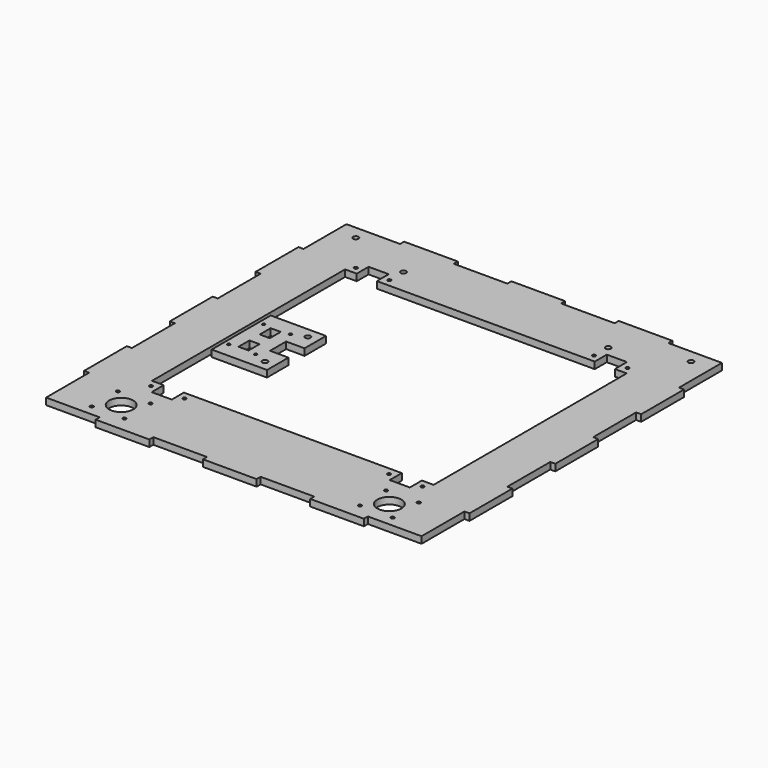
from build123d import *

# Parameters (mm, degrees)
F0_R     = 1.5875
F0_R_2   = 11.43
F0_R_3   = 3.175
F0_W     = 4.7625
F0_H     = 50.8
F0_W_2   = 50.8
F0_H_2   = 4.7625
F0_W_3   = 44.45
F0_H_3   = 41.1268851364
F1_DEPTH = 6.35
F0_R_4   = 1.8415
F0_W_4   = 9.525
F0_H_4   = 12.954
F2_D     = 2.7051
F3_D     = 5.1054
F4_D     = 5.1054


with BuildPart() as f1:
    # F0 (on Top) → F1 (new body)
    with BuildSketch(Plane.XY):
        with BuildLine():
            ThreePointArc((155.575, 171.45), (158.75, 174.625), (161.925, 171.45))
            Line((161.925, 171.45), (177.8, 171.45))
            Line((177.8, 171.45), (177.8, 184.15))
            Line((177.8, 184.15), (127, 184.15))
            Line((127, 184.15), (76.2, 184.15))
            Line((76.2, 184.15), (25.4, 184.15))
            Line((25.4, 184.15), (-25.4, 184.15))
            Line((-25.4, 184.15), (-76.2, 184.15))
            Line((-76.2, 184.15), (-127, 184.15))
            Line((-127, 184.15), (-177.8, 184.15))
            Line((-177.8, 184.15), (-177.8, 171.45))
            Line((-177.8, 171.45), (-161.925, 171.45))
            ThreePointArc((-161.925, 171.45), (-158.75, 174.625), (-155.575, 171.45))
            Line((-155.575, 171.45), (155.575, 171.45))
        make_face()
        with BuildLine():
            ThreePointArc((155.575, 171.45), (158.75, 168.275), (161.925, 171.45))
            Line((161.925, 171.45), (155.575, 171.45))
        make_face()
        with BuildLine():
            Line((155.575, 171.45), (161.925, 171.45))
            ThreePointArc((161.925, 171.45), (158.75, 174.625), (155.575, 171.45))
        make_face()
        with BuildLine():
            Line((177.8, 171.45), (161.925, 171.45))
            ThreePointArc((161.925, 171.45), (158.75, 168.275), (155.575, 171.45))
            Line((155.575, 171.45), (-155.575, 171.45))
            ThreePointArc((-155.575, 171.45), (-158.75, 168.275), (-161.925, 171.45))
            Line((-161.925, 171.45), (-177.8, 171.45))
            Line((-177.8, 171.45), (-177.8, 133.35))
            Line((-177.8, 133.35), (-177.8, 82.55))
            Line((-177.8, 82.55), (-177.8, 31.75))
            Line((-177.8, 31.75), (-177.8, -19.05))
            Line((-177.8, -19.05), (-177.8, -69.85))
            Line((-177.8, -69.85), (-177.8, -120.65))
            Line((-177.8, -120.65), (-177.8, -171.45))
            Line((-177.8, -171.45), (-127, -171.45))
            Line((-127, -171.45), (-76.2, -171.45))
            Line((-76.2, -171.45), (-25.4, -171.45))
            Line((-25.4, -171.45), (25.4, -171.45))
            Line((25.4, -171.45), (76.2, -171.45))
            Line((76.2, -171.45), (127, -171.45))
            Line((127, -171.45), (177.8, -171.45))
            Line((177.8, -171.45), (177.8, -120.65))
            Line((177.8, -120.65), (177.8, -69.85))
            Line((177.8, -69.85), (177.8, -19.05))
            Line((177.8, -19.05), (177.8, 31.75))
            Line((177.8, 31.75), (177.8, 82.55))
            Line((177.8, 82.55), (177.8, 133.35))
            Line((177.8, 133.35), (177.8, 171.45))
        make_face()
        with Locations((-142.494, -161.544)):
            Circle(F0_R, mode=Mode.SUBTRACT)
        with Locations((-111.506, -161.544)):
            Circle(F0_R, mode=Mode.SUBTRACT)
        with Locations((-127, -146.05)):
            Circle(F0_R_2, mode=Mode.SUBTRACT)
        with Locations((-142.494, -130.556)):
            Circle(F0_R, mode=Mode.SUBTRACT)
        with Locations((-128.5875, -108.7501)):
            Circle(F0_R, mode=Mode.SUBTRACT)
        with Locations((-111.506, -130.556)):
            Circle(F0_R, mode=Mode.SUBTRACT)
        with Locations((-96.8375, -108.7501)):
            Circle(F0_R, mode=Mode.SUBTRACT)
        with Locations((111.506, -161.544)):
            Circle(F0_R, mode=Mode.SUBTRACT)
        with Locations((127, -146.05)):
            Circle(F0_R_2, mode=Mode.SUBTRACT)
        with Locations((142.494, -161.544)):
            Circle(F0_R, mode=Mode.SUBTRACT)
        with Locations((111.506, -130.556)):
            Circle(F0_R, mode=Mode.SUBTRACT)
        with Locations((96.8375, -108.7501)):
            Circle(F0_R, mode=Mode.SUBTRACT)
        with Locations((128.5875, -108.7501)):
            Circle(F0_R, mode=Mode.SUBTRACT)
        with Locations((142.494, -130.556)):
            Circle(F0_R, mode=Mode.SUBTRACT)
        with Locations((-128.7030479432, 133.9005806915)):
            Circle(F0_R, mode=Mode.SUBTRACT)
        with Locations((-96.9530623423, 133.9308187798)):
            Circle(F0_R, mode=Mode.SUBTRACT)
        with Locations((-96.9530623423, 150.6059263422)):
            Circle(F0_R_3, mode=Mode.SUBTRACT)
        Polygon((-122.2375, -101.6), (-133.35, -101.6), (-133.35, 126.7460517791), (-133.35, 127), (-122.3464730803, 127), (-122.3598604405, 141.0567250665), (-103.30986908, 141.0748679195), (-103.2964644408, 127), (-22.225, 127), (-22.225, 168.1268851364), (22.225, 168.1268851364), (22.225, 127), (103.0786291533, 127), (103.065037326, 141.271415494), (122.1150286865, 141.289558347), (122.1286377928, 127), (133.2411428818, 127), (133.35, 127), (133.35, -101.6), (122.2375, -101.6), (122.2375, -115.9002), (103.1875, -115.9002), (103.1875, -101.6), (-103.1875, -101.6), (-103.1875, -115.9002), (-122.2375, -115.9002), align=None, mode=Mode.SUBTRACT)
        with Locations((96.7218498233, 134.115271119)):
            Circle(F0_R, mode=Mode.SUBTRACT)
        with Locations((128.4718354242, 134.1455092073)):
            Circle(F0_R, mode=Mode.SUBTRACT)
        with Locations((96.9530623423, 150.6059263422)):
            Circle(F0_R_3, mode=Mode.SUBTRACT)
        with Locations((180.18125, 107.95)):
            Rectangle(F0_W, F0_H)
        with BuildLine():
            ThreePointArc((-161.925, 171.45), (-158.75, 168.275), (-155.575, 171.45))
            Line((-155.575, 171.45), (-161.925, 171.45))
        make_face()
        with BuildLine():
            Line((-161.925, 171.45), (-155.575, 171.45))
            ThreePointArc((-155.575, 171.45), (-158.75, 174.625), (-161.925, 171.45))
        make_face()
        with Locations((101.6, 186.53125)):
            Rectangle(F0_W_2, F0_H_2)
        with Locations((180.18125, 6.35)):
            Rectangle(F0_W, F0_H)
        with Locations((0, 186.53125)):
            Rectangle(F0_W_2, F0_H_2)
        with Locations((-180.18125, 107.95)):
            Rectangle(F0_W, F0_H)
        with Locations((180.18125, -95.25)):
            Rectangle(F0_W, F0_H)
        with Locations((-101.6, 186.53125)):
            Rectangle(F0_W_2, F0_H_2)
        with Locations((-180.18125, 6.35)):
            Rectangle(F0_W, F0_H)
        with Locations((101.6, -173.83125)):
            Rectangle(F0_W_2, F0_H_2)
        with Locations((-180.18125, -95.25)):
            Rectangle(F0_W, F0_H)
        with Locations((0, -173.83125)):
            Rectangle(F0_W_2, F0_H_2)
        with Locations((-101.6, -173.83125)):
            Rectangle(F0_W_2, F0_H_2)
        with Locations((0, 147.5634425682)):
            Rectangle(F0_W_3, F0_H_3)
        with Locations((-96.9530623423, 150.6059263422)):
            Circle(F0_R_3)
        with Locations((96.9530623423, 150.6059263422)):
            Circle(F0_R_3)
    extrude(amount=F1_DEPTH)

    # F4 (through all)
    with Locations(Plane(origin=(0, 0, 0), x_dir=(1, 0, 0), z_dir=(0, 0, -1))):
        with Locations((-158.75, -171.45), (-96.9530623423, -150.6059263422), (96.9530623423, -150.6059263422), (158.75, -171.45)):
            Hole(F4_D / 2)


with BuildPart() as f1b:
    # F0 (on Top) → F1, piece 2 (new body)
    with BuildSketch(Plane.XY):
        with BuildLine():
            Line((-130.175, 34.925), (-130.175, 25.4))
            Line((-130.175, 25.4), (-95.25, 25.4))
            Line((-95.25, 25.4), (-90.4875, 25.4))
            ThreePointArc((-90.4875, 25.4), (-87.3125, 28.575), (-84.1375, 25.4))
            Line((-84.1375, 25.4), (-77.7875, 25.4))
            Line((-77.7875, 25.4), (-77.7875, 34.925))
            Line((-77.7875, 34.925), (-100.0125, 34.925))
            Line((-100.0125, 34.925), (-130.175, 34.925))
        make_face()
        Polygon((-95.25, 25.4), (-130.175, 25.4), (-130.175, -25.4), (-95.25, -25.4), (-95.25, -9.525), (-95.25, 9.525), align=None)
        with Locations((-125.4125, -20.6375)):
            Circle(F0_R_4, mode=Mode.SUBTRACT)
        with Locations((-100.0125, -20.6375)):
            Circle(F0_R_4, mode=Mode.SUBTRACT)
        with Locations((-112.7125, -12.573)):
            Rectangle(F0_W_4, F0_H_4, mode=Mode.SUBTRACT)
        with Locations((-125.4125, 20.6375)):
            Circle(F0_R_4, mode=Mode.SUBTRACT)
        with Locations((-112.7125, 12.573)):
            Rectangle(F0_W_4, F0_H_4, mode=Mode.SUBTRACT)
        with Locations((-100.0125, 20.6375)):
            Circle(F0_R_4, mode=Mode.SUBTRACT)
        with BuildLine():
            Line((-90.4875, 25.4), (-95.25, 25.4))
            Line((-95.25, 25.4), (-95.25, 9.525))
            Line((-95.25, 9.525), (-77.7875, 9.525))
            Line((-77.7875, 9.525), (-77.7875, 25.4))
            Line((-77.7875, 25.4), (-84.1375, 25.4))
            ThreePointArc((-84.1375, 25.4), (-87.3125, 22.225), (-90.4875, 25.4))
        make_face()
        with BuildLine():
            Line((-95.25, -25.4), (-130.175, -25.4))
            Line((-130.175, -25.4), (-130.175, -34.925))
            Line((-130.175, -34.925), (-100.0125, -34.925))
            Line((-100.0125, -34.925), (-77.7875, -34.925))
            Line((-77.7875, -34.925), (-77.7875, -25.4))
            Line((-77.7875, -25.4), (-84.1375, -25.4))
            ThreePointArc((-84.1375, -25.4), (-87.3125, -28.575), (-90.4875, -25.4))
            Line((-90.4875, -25.4), (-95.25, -25.4))
        make_face()
        with BuildLine():
            ThreePointArc((-84.1375, 25.4), (-87.3125, 28.575), (-90.4875, 25.4))
            Line((-90.4875, 25.4), (-84.1375, 25.4))
        make_face()
        with BuildLine():
            Line((-84.1375, 25.4), (-90.4875, 25.4))
            ThreePointArc((-90.4875, 25.4), (-87.3125, 22.225), (-84.1375, 25.4))
        make_face()
        with BuildLine():
            Line((-95.25, -9.525), (-95.25, -25.4))
            Line((-95.25, -25.4), (-90.4875, -25.4))
            ThreePointArc((-90.4875, -25.4), (-87.3125, -22.225), (-84.1375, -25.4))
            Line((-84.1375, -25.4), (-77.7875, -25.4))
            Line((-77.7875, -25.4), (-77.7875, -9.525))
            Line((-77.7875, -9.525), (-95.25, -9.525))
        make_face()
        with BuildLine():
            ThreePointArc((-84.1375, -25.4), (-87.3125, -22.225), (-90.4875, -25.4))
            Line((-90.4875, -25.4), (-84.1375, -25.4))
        make_face()
        with BuildLine():
            Line((-84.1375, -25.4), (-90.4875, -25.4))
            ThreePointArc((-90.4875, -25.4), (-87.3125, -28.575), (-84.1375, -25.4))
        make_face()
        with Locations((-125.4125, 20.6375)):
            Circle(F0_R_4)
        with Locations((-100.0125, 20.6375)):
            Circle(F0_R_4)
        with Locations((-125.4125, -20.6375)):
            Circle(F0_R_4)
        with Locations((-100.0125, -20.6375)):
            Circle(F0_R_4)
    extrude(amount=F1_DEPTH)

    # F2 (through all)
    with Locations(Plane(origin=(0, 0, 0), x_dir=(1, 0, 0), z_dir=(0, 0, -1))):
        with Locations((-125.4125, -20.6375), (-100.0125, -20.6375), (-100.0125, 20.6375), (-125.4125, 20.6375)):
            Hole(F2_D / 2)

    # F3 (through all)
    with Locations(Plane(origin=(0, 0, 0), x_dir=(1, 0, 0), z_dir=(0, 0, -1))):
        with Locations((-87.3125, -25.4), (-87.3125, 25.4)):
            Hole(F3_D / 2)


solid = Compound([f1.part, f1b.part])
